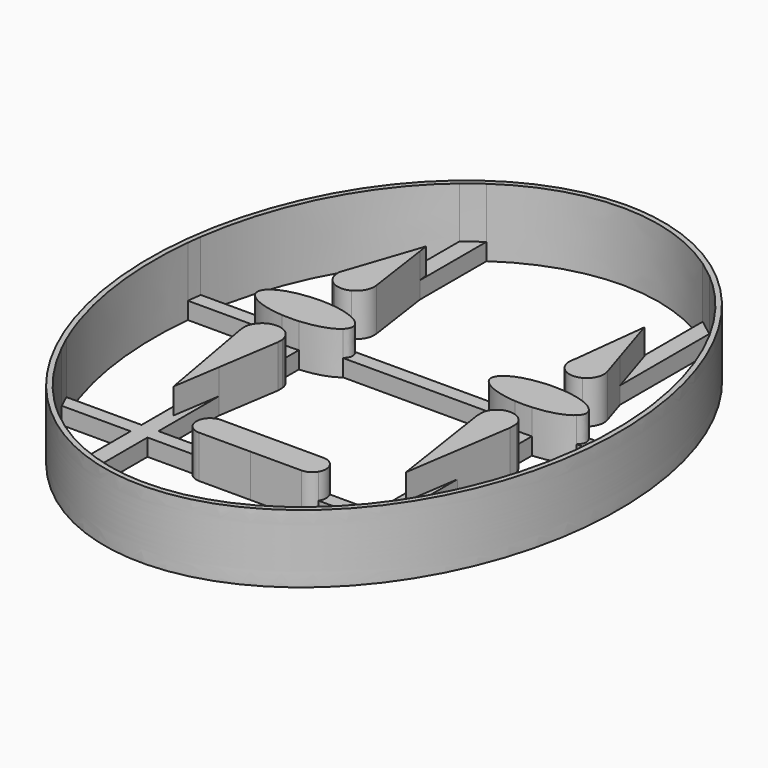
from build123d import *

# Parameters (mm, degrees)
F1_DEPTH = 10.16
F2_DEPTH = 6.35
F3_DEPTH = 2.54


# Not quite as in the source:
# - the dataset's text gives a spline's control points without its knots; the knots are read off the source's solid


with BuildPart() as f1:
    # F0 (on Top) → F1 (new body)
    with BuildSketch(Plane.XY):
        with BuildLine():
            add(Edge.make_bspline(
                [(0.8874152158, 46.7860518305), (0.3035465665, 46.7860518305), (-0.8641907321, 46.7484087934), (-3.1804804426, 46.524648738), (-6.0388714179, 45.9705936493), (-9.3828884747, 44.8801852683), (-12.6174065606, 43.3780630031), (-15.7189563215, 41.4780777699), (-18.6646785296, 39.1941395739), (-20.9712493188, 36.9817445808), (-22.7157476895, 35.0339858624), (-23.9729196354, 33.4833733883), (-25.1682601082, 31.8548035031), (-26.6676910685, 29.5980430053), (-28.3672543912, 26.6201447797), (-30.1171589074, 22.8270664956), (-31.5692954578, 18.84316303), (-32.7148026715, 14.6976460619), (-33.5447958259, 10.419700464), (-33.965961995, 6.767927242), (-34.135986765, 3.8102925283), (-34.1788837939, 1.5740518305), (-34.135986765, -0.6621888672), (-33.965961995, -3.619823581), (-33.5447958259, -7.271596803), (-32.7148026715, -11.5495424009), (-31.5692954578, -15.6950593689), (-30.1171589074, -19.6789628346), (-28.3672543912, -23.4720411187), (-26.6676910685, -26.4499393442), (-25.1682601082, -28.7066998421), (-23.9729196354, -30.3352697272), (-22.7157476895, -31.8858822014), (-20.9712493188, -33.8336409198), (-18.6646785296, -36.0460359129), (-15.7189563215, -38.3299741089), (-12.6174065606, -40.2299593421), (-9.3828884747, -41.7320816073), (-6.0388714179, -42.8224899883), (-3.1804804426, -43.376545077), (-0.8641907321, -43.6003051324), (0.8874152158, -43.656769688), (2.6390211637, -43.6003051324), (4.9553108741, -43.376545077), (7.8137018494, -42.8224899883), (11.1577189062, -41.7320816073), (14.3922369922, -40.2299593421), (17.493786753, -38.3299741089), (20.4395089612, -36.0460359129), (22.7460797504, -33.8336409198), (24.490578121, -31.8858822014), (25.7477500669, -30.3352697272), (26.9430905397, -28.7066998421), (28.4425215001, -26.4499393442), (30.1420848227, -23.4720411187), (31.8919893389, -19.6789628346), (33.3441258894, -15.6950593689), (34.489633103, -11.5495424009), (35.3196262574, -7.271596803), (35.7407924266, -3.619823581), (35.9108171965, -0.6621888672), (35.9537142254, 1.5740518305), (35.9108171965, 3.8102925283), (35.7407924266, 6.767927242), (35.3196262574, 10.419700464), (34.489633103, 14.6976460619), (33.3441258894, 18.84316303), (31.8919893389, 22.8270664956), (30.1420848227, 26.6201447797), (28.4425215001, 29.5980430053), (26.9430905397, 31.8548035031), (25.7477500669, 33.4833733883), (24.490578121, 35.0339858624), (22.7460797504, 36.9817445808), (20.4395089612, 39.1941395739), (17.493786753, 41.4780777699), (14.3922369922, 43.3780630031), (11.1577189062, 44.8801852683), (7.8137018494, 45.9705936493), (4.9553108741, 46.524648738), (2.6390211637, 46.7484087934), (1.4712838651, 46.7860518305), (0.8874152158, 46.7860518305)],
                knots=[0, 0, 0, 0, 0.0078125, 0.015625, 0.03125, 0.046875, 0.0625, 0.078125, 0.09375, 0.109375, 0.1171875, 0.125, 0.1328125, 0.140625, 0.15625, 0.171875, 0.1875, 0.203125, 0.21875, 0.234375, 0.2421875, 0.25, 0.2578125, 0.265625, 0.28125, 0.296875, 0.3125, 0.328125, 0.34375, 0.359375, 0.3671875, 0.375, 0.3828125, 0.390625, 0.40625, 0.421875, 0.4375, 0.453125, 0.46875, 0.484375, 0.4921875, 0.5, 0.5078125, 0.515625, 0.53125, 0.546875, 0.5625, 0.578125, 0.59375, 0.609375, 0.6171875, 0.625, 0.6328125, 0.640625, 0.65625, 0.671875, 0.6875, 0.703125, 0.71875, 0.734375, 0.7421875, 0.75, 0.7578125, 0.765625, 0.78125, 0.796875, 0.8125, 0.828125, 0.84375, 0.859375, 0.8671875, 0.875, 0.8828125, 0.890625, 0.90625, 0.921875, 0.9375, 0.953125, 0.96875, 0.984375, 0.9921875, 1, 1, 1, 1], degree=3))
        make_face()
        with BuildLine():
            add(Edge.make_bspline(
                [(0.8874152158, 46.0240518305), (-7.6730270574, 46.0240518305), (-15.2290235078, 40.8084782188)],
                knots=[0, 0, 0, 0.4892953614, 0.4892953614, 0.4892953614], degree=2, weights=[1, 0.970222722, 1]))
            add(Edge.make_bspline(
                [(17.0038539393, 40.8084782188), (9.447857489, 46.0240518305), (0.8874152158, 46.0240518305)],
                knots=[5.7938899458, 5.7938899458, 5.7938899458, 6.2831853072, 6.2831853072, 6.2831853072], degree=2, weights=[1, 0.970222722, 1]))
            add(Edge.make_bspline(
                [(19.5227909328, 38.8868294251), (18.2949402613, 39.9172978436), (17.0038539393, 40.8084782188)],
                knots=[5.7086272545, 5.7086272545, 5.7086272545, 5.7938899458, 5.7938899458, 5.7938899458], degree=2, weights=[1, 0.9990914218, 1]))
            add(Edge.make_bspline(
                [(34.6163309811, 9.5822196506), (31.9493168533, 28.457920756), (19.5227909328, 38.8868294251)],
                knots=[4.8935393675, 4.8935393675, 4.8935393675, 5.7086272545, 5.7086272545, 5.7086272545], degree=2, weights=[1, 0.9180970627, 1]))
            add(Edge.make_bspline(
                [(34.8708896875, 7.5041735472), (34.7625862899, 8.5471027136), (34.6163309811, 9.5822196506)],
                knots=[4.8461989994, 4.8461989994, 4.8461989994, 4.8935393675, 4.8935393675, 4.8935393675], degree=2, weights=[1, 0.9997198743, 1]))
            add(Edge.make_bspline(
                [(30.7375906283, -20.3011595258), (36.408100645, -7.2987059431), (34.8708896875, 7.5041735472)],
                knots=[4.1978532573, 4.1978532573, 4.1978532573, 4.8461989994, 4.8461989994, 4.8461989994], degree=2, weights=[1, 0.9479145118, 1]))
            add(Edge.make_bspline(
                [(29.7867641343, -22.3506663998), (30.2834517092, -21.3424979944), (30.7375906283, -20.3011595258)],
                knots=[4.1440428934, 4.1440428934, 4.1440428934, 4.1978532573, 4.1978532573, 4.1978532573], degree=2, weights=[1, 0.9996380774, 1]))
            add(Edge.make_bspline(
                [(19.5227909328, -35.7387257641), (25.7767590963, -30.490109762), (29.7867641343, -22.3506663998)],
                knots=[3.7161507062, 3.7161507062, 3.7161507062, 4.1440428934, 4.1440428934, 4.1440428934], degree=2, weights=[1, 0.9772006998, 1]))
            add(Edge.make_bspline(
                [(17.0038539393, -37.6603745577), (18.2949402613, -36.7691941826), (19.5227909328, -35.7387257641)],
                knots=[3.630888015, 3.630888015, 3.630888015, 3.7161507062, 3.7161507062, 3.7161507062], degree=2, weights=[1, 0.9990914218, 1]))
            add(Edge.make_bspline(
                [(-15.2290235078, -37.6603745577), (0.8874152158, -48.7848467666), (17.0038539393, -37.6603745577)],
                knots=[2.6522972922, 2.6522972922, 2.6522972922, 3.630888015, 3.630888015, 3.630888015], degree=2, weights=[1, 0.8826642607, 1]))
            add(Edge.make_bspline(
                [(-17.7479605013, -35.7387257641), (-16.5201098298, -36.7691941826), (-15.2290235078, -37.6603745577)],
                knots=[2.5670346009, 2.5670346009, 2.5670346009, 2.6522972922, 2.6522972922, 2.6522972922], degree=2, weights=[1, 0.9990914218, 1]))
            add(Edge.make_bspline(
                [(-28.0119337027, -22.3506663998), (-24.0019286648, -30.490109762), (-17.7479605013, -35.7387257641)],
                knots=[2.1391424138, 2.1391424138, 2.1391424138, 2.5670346009, 2.5670346009, 2.5670346009], degree=2, weights=[1, 0.9772006998, 1]))
            add(Edge.make_bspline(
                [(-28.9627601968, -20.3011595258), (-28.5086212776, -21.3424979944), (-28.0119337027, -22.3506663998)],
                knots=[2.0853320499, 2.0853320499, 2.0853320499, 2.1391424138, 2.1391424138, 2.1391424138], degree=2, weights=[1, 0.9996380774, 1]))
            add(Edge.make_bspline(
                [(-33.096059256, 7.5041735472), (-34.6332702135, -7.2987059431), (-28.9627601968, -20.3011595258)],
                knots=[1.4369863078, 1.4369863078, 1.4369863078, 2.0853320499, 2.0853320499, 2.0853320499], degree=2, weights=[1, 0.9479145118, 1]))
            add(Edge.make_bspline(
                [(-32.8415005495, 9.5822196506), (-32.9877558584, 8.5471027136), (-33.096059256, 7.5041735472)],
                knots=[1.3896459397, 1.3896459397, 1.3896459397, 1.4369863078, 1.4369863078, 1.4369863078], degree=2, weights=[1, 0.9997198743, 1]))
            add(Edge.make_bspline(
                [(-17.7479605013, 38.8868294251), (-30.1744864217, 28.457920756), (-32.8415005495, 9.5822196506)],
                knots=[0.5745580526, 0.5745580526, 0.5745580526, 1.3896459397, 1.3896459397, 1.3896459397], degree=2, weights=[1, 0.9180970627, 1]))
            add(Edge.make_bspline(
                [(-15.2290235078, 40.8084782188), (-16.5201098298, 39.9172978436), (-17.7479605013, 38.8868294251)],
                knots=[0.4892953614, 0.4892953614, 0.4892953614, 0.5745580526, 0.5745580526, 0.5745580526], degree=2, weights=[1, 0.9990914218, 1]))
        make_face(mode=Mode.SUBTRACT)
    extrude(amount=F1_DEPTH)



with BuildPart() as f2:
    # F0 (on Top) → F2 (new body)
    with BuildSketch(Plane.XY):
        with BuildLine():
            add(Edge.make_bspline(
                [(-17.7479605013, 11.44730103), (-21.8523231253, 11.159864588), (-23.2315880612, 9.5822196506)],
                knots=[4.88516773, 4.88516773, 4.88516773, 5.9457744715, 5.9457744715, 5.9457744715], degree=2, weights=[1, 0.8626536668, 1]))
            add(Edge.make_bspline(
                [(-23.2315880612, 9.5822196506), (-23.6322576844, 9.1239216208), (-23.6322576844, 8.6382383173)],
                knots=[5.9457744715, 5.9457744715, 5.9457744715, 6.2831853072, 6.2831853072, 6.2831853072], degree=2, weights=[1, 0.9858029614, 1]))
            add(Edge.make_bspline(
                [(-23.6322576844, 8.6382383173), (-23.6322576844, 8.0468135504), (-23.0461097972, 7.5041735472)],
                knots=[0, 0, 0, 0.4090146334, 0.4090146334, 0.4090146334], degree=2, weights=[1, 0.9791611598, 1]))
            add(Edge.make_bspline(
                [(-23.0461097972, 7.5041735472), (-21.522333432, 6.093502231), (-17.7479605013, 5.8291756045)],
                knots=[0.4090146334, 0.4090146334, 0.4090146334, 1.3980175772, 1.3980175772, 1.3980175772], degree=2, weights=[1, 0.8802054171, 1]))
            add(Edge.make_bspline(
                [(-17.7479605013, 5.8291756045), (-16.4872656687, 5.7408867104), (-15.2290235078, 5.8346406134)],
                knots=[1.3980175772, 1.3980175772, 1.3980175772, 1.7543880589, 1.7543880589, 1.7543880589], degree=2, weights=[1, 0.9841669681, 1]))
            add(Edge.make_bspline(
                [(-15.2290235078, 5.8346406134), (-11.5106062448, 6.1117066203), (-10.0064938636, 7.5041735472)],
                knots=[1.7543880589, 1.7543880589, 1.7543880589, 2.7325780202, 2.7325780202, 2.7325780202], degree=2, weights=[1, 0.8827584227, 1]))
            add(Edge.make_bspline(
                [(-10.0064938636, 7.5041735472), (-8.8999042079, 8.5286245899), (-9.8210155996, 9.5822196506)],
                knots=[2.7325780202, 2.7325780202, 2.7325780202, 3.4790034893, 3.4790034893, 3.4790034893], degree=2, weights=[1, 0.9311607616, 1]))
            add(Edge.make_bspline(
                [(-9.8210155996, 9.5822196506), (-11.1832439782, 11.1403776587), (-15.2290235078, 11.4418360212)],
                knots=[3.4790034893, 3.4790034893, 3.4790034893, 4.5287972483, 4.5287972483, 4.5287972483], degree=2, weights=[1, 0.8653756223, 1]))
            add(Edge.make_bspline(
                [(-15.2290235078, 11.4418360212), (-16.4872656687, 11.5355899242), (-17.7479605013, 11.44730103)],
                knots=[4.5287972483, 4.5287972483, 4.5287972483, 4.88516773, 4.88516773, 4.88516773], degree=2, weights=[1, 0.9841669681, 1]))
        make_face()
    extrude(amount=F2_DEPTH)


with BuildPart() as f2b:
    # F0 (on Top) → F2, piece 2 (new body)
    with BuildSketch(Plane.XY):
        with BuildLine():
            Line((-13.8026518037, 18.5152967152), (-15.2290235078, 28.4465199794))
            Line((-15.2290235078, 28.4465199794), (-15.4276108953, 29.8292000182))
            Line((-15.4276108953, 29.8292000182), (-17.7479605013, 22.9402716964))
            Line((-17.7479605013, 22.9402716964), (-19.2382517874, 18.5157186799))
            ThreePointArc((-19.2382517874, 18.5157186799), (-18.953046125, 16.8515255575), (-17.7479605013, 15.6688803622))
            ThreePointArc((-17.7479605013, 15.6688803622), (-16.4844803046, 15.3794653342), (-15.2290235078, 15.7019114496))
            ThreePointArc((-15.2290235078, 15.7019114496), (-14.0715265067, 16.8833406396), (-13.8026518037, 18.5152967152))
        make_face()
    extrude(amount=F2_DEPTH)


with BuildPart() as f2c:
    # F0 (on Top) → F2, piece 3 (new body)
    with BuildSketch(Plane.XY):
        with BuildLine():
            Line((17.1461113686, 29.7382220353), (17.0038539393, 28.497185345))
            Line((17.0038539393, 28.497185345), (15.8444382697, 18.382582593))
            ThreePointArc((15.8444382697, 18.382582593), (15.8857831263, 16.6578406118), (17.0038539393, 15.3439296727))
            ThreePointArc((17.0038539393, 15.3439296727), (18.2581575627, 14.9961423132), (19.5227909328, 15.3042592817))
            ThreePointArc((19.5227909328, 15.3042592817), (20.6927393028, 16.6091812711), (20.7603491707, 18.3604749337))
            Line((20.7603491707, 18.3604749337), (19.5227909328, 22.2563515817))
            Line((19.5227909328, 22.2563515817), (17.1461113686, 29.7382220353))
        make_face()
    extrude(amount=F2_DEPTH)


with BuildPart() as f2d:
    # F0 (on Top) → F2, piece 4 (new body)
    with BuildSketch(Plane.XY):
        with BuildLine():
            add(Edge.make_bspline(
                [(25.4135646224, 8.6382383173), (25.4135646224, 9.1239216208), (25.0128949991, 9.5822196506)],
                knots=[0, 0, 0, 0.3374108357, 0.3374108357, 0.3374108357], degree=2, weights=[1, 0.9858029614, 1]))
            add(Edge.make_bspline(
                [(25.0128949991, 9.5822196506), (23.632167473, 11.1615375429), (19.5227909328, 11.4477533536)],
                knots=[0.3374108357, 0.3374108357, 0.3374108357, 1.3989426975, 1.3989426975, 1.3989426975], degree=2, weights=[1, 0.8624196139, 1]))
            add(Edge.make_bspline(
                [(19.5227909328, 11.4477533536), (18.2618860231, 11.5355746855), (17.0038539393, 11.4413521986)],
                knots=[1.3989426975, 1.3989426975, 1.3989426975, 1.7553151371, 1.7553151371, 1.7553151371], degree=2, weights=[1, 0.9841667946, 1]))
            add(Edge.make_bspline(
                [(17.0038539393, 11.4413521986), (12.9630952221, 11.1387125918), (11.6023225375, 9.5822196506)],
                knots=[1.7553151371, 1.7553151371, 1.7553151371, 2.8041818179, 2.8041818179, 2.8041818179], degree=2, weights=[1, 0.8656078198, 1]))
            add(Edge.make_bspline(
                [(11.6023225375, 9.5822196506), (10.6812111458, 8.5286245899), (11.7878008015, 7.5041735472)],
                knots=[2.8041818179, 2.8041818179, 2.8041818179, 3.5506072869, 3.5506072869, 3.5506072869], degree=2, weights=[1, 0.9311607616, 1]))
            add(Edge.make_bspline(
                [(11.7878008015, 7.5041735472), (13.2902325239, 6.1132625292), (17.0038539393, 5.8351244359)],
                knots=[3.5506072869, 3.5506072869, 3.5506072869, 4.5278701701, 4.5278701701, 4.5278701701], degree=2, weights=[1, 0.8829761111, 1]))
            add(Edge.make_bspline(
                [(17.0038539393, 5.8351244359), (18.2618860231, 5.7409019491), (19.5227909328, 5.828723281)],
                knots=[4.5278701701, 4.5278701701, 4.5278701701, 4.8842426097, 4.8842426097, 4.8842426097], degree=2, weights=[1, 0.9841667946, 1]))
            add(Edge.make_bspline(
                [(19.5227909328, 5.828723281), (23.3019526806, 6.0919398134), (24.8274167351, 7.5041735472)],
                knots=[4.8842426097, 4.8842426097, 4.8842426097, 5.8741706738, 5.8741706738, 5.8741706738], degree=2, weights=[1, 0.8799857952, 1]))
            add(Edge.make_bspline(
                [(24.8274167351, 7.5041735472), (25.4135646224, 8.0468135504), (25.4135646224, 8.6382383173)],
                knots=[5.8741706738, 5.8741706738, 5.8741706738, 6.2831853072, 6.2831853072, 6.2831853072], degree=2, weights=[1, 0.9791611598, 1]))
        make_face()
    extrude(amount=F2_DEPTH)


with BuildPart() as f2e:
    # F0 (on Top) → F2, piece 5 (new body)
    with BuildSketch(Plane.XY):
        with BuildLine():
            Line((18.3088215866, -16.1279799693), (19.5227909328, -8.0577728991))
            Line((19.5227909328, -8.0577728991), (20.7629566947, 0.1865823074))
            Line((20.7629566947, 0.1865823074), (20.7627794612, 1.4218628216))
            ThreePointArc((20.7627794612, 1.4218628216), (20.3102626812, 2.3535523253), (19.5227909328, 3.0263858953))
            ThreePointArc((19.5227909328, 3.0263858953), (18.9347962572, 3.2586504045), (18.3076087683, 3.3381513144))
            Line((18.3076087683, 3.3381513144), (18.3023937202, 3.3381513144))
            ThreePointArc((18.3023937202, 3.3381513144), (17.6287933652, 3.2462728126), (17.0038539393, 2.9786353503))
            ThreePointArc((17.0038539393, 2.9786353503), (16.2672974346, 2.3106387051), (15.8444382697, 1.4106803009))
            Line((15.8444382697, 1.4106803009), (15.8444382697, 0.1970595365))
            Line((15.8444382697, 0.1970595365), (17.0038539393, -7.4833635861))
            Line((17.0038539393, -7.4833635861), (18.3088215866, -16.1279799693))
        make_face()
    extrude(amount=F2_DEPTH)


with BuildPart() as f2f:
    # F0 (on Top) → F2, piece 6 (new body)
    with BuildSketch(Plane.XY):
        with BuildLine():
            Line((-19.2441018304, 0.1865863317), (-17.7479605013, -8.1779694256))
            Line((-17.7479605013, -8.1779694256), (-16.3255312883, -16.1304189912))
            Line((-16.3255312883, -16.1304189912), (-15.2290235078, -9.0221496637))
            Line((-15.2290235078, -9.0221496637), (-13.8085018304, 0.1865863317))
            Line((-13.8085018304, 0.1865863317), (-13.8085018304, 1.0250714))
            ThreePointArc((-13.8085018304, 1.0250714), (-14.2822654949, 2.195326292), (-15.2290235078, 3.0305494881))
            ThreePointArc((-15.2290235078, 3.0305494881), (-15.7076702442, 3.2310990364), (-16.2154720062, 3.3381513144))
            Line((-16.2154720062, 3.3381513144), (-16.5263018304, 3.3381513144))
            Line((-16.5263018304, 3.3381513144), (-16.8371316545, 3.3381513144))
            ThreePointArc((-16.8371316545, 3.3381513144), (-17.304229567, 3.2434470298), (-17.7479605013, 3.0695153788))
            ThreePointArc((-17.7479605013, 3.0695153788), (-18.745484439, 2.2298453965), (-19.2441018304, 1.0250714))
            Line((-19.2441018304, 1.0250714), (-19.2441018304, 0.1865863317))
        make_face()
    extrude(amount=F2_DEPTH)


with BuildPart() as f2g:
    # F0 (on Top) → F2, piece 7 (new body)
    with BuildSketch(Plane.XY):
        with BuildLine():
            ThreePointArc((-8.5105954788, -20.3011595258), (-8.7762969648, -21.3283492866), (-8.4924240981, -22.3506663998))
            ThreePointArc((-8.4924240981, -22.3506663998), (-7.7440409154, -23.088748383), (-6.7281162348, -23.3584508958))
            Line((-6.7281162348, -23.3584508958), (0.8933992052, -23.3584508958))
            Line((0.8933992052, -23.3584508958), (8.5133986834, -23.355631034))
            ThreePointArc((8.5133986834, -23.355631034), (9.527123423, -23.0865386285), (10.2744791839, -22.3506663998))
            ThreePointArc((10.2744791839, -22.3506663998), (10.5593969681, -21.3285723586), (10.2942984138, -20.3011595258))
            ThreePointArc((10.2942984138, -20.3011595258), (9.5436122613, -19.5405321417), (8.5118837652, -19.2619284317))
            Line((8.5118837652, -19.2619284317), (0.8918837652, -19.2619284317))
            Line((0.8918837652, -19.2619284317), (-6.7281162348, -19.2619284317))
            ThreePointArc((-6.7281162348, -19.2619284317), (-7.7597694616, -19.5407079051), (-8.5105954788, -20.3011595258))
        make_face()
    extrude(amount=F2_DEPTH)


with BuildPart() as f1_1:
    add(f1.part)

    add(f2.part)  # F3 merges F2

    add(f2b.part)  # F3 merges F2b

    add(f2c.part)  # F3 merges F2c

    add(f2d.part)  # F3 merges F2d

    add(f2e.part)  # F3 merges F2e

    add(f2f.part)  # F3 merges F2f

    add(f2g.part)  # F3 merges F2g
    # F0 (on Top) → F3 (join)
    with BuildSketch(Plane.XY):
        with BuildLine():
            ThreePointArc((19.5227909328, 15.3042592817), (18.2581575627, 14.9961423132), (17.0038539393, 15.3439296727))
            Line((17.0038539393, 15.3439296727), (17.0038539393, 11.4413521986))
            add(Edge.make_bspline(
                [(19.5227909328, 11.4477533536), (18.2618860231, 11.5355746855), (17.0038539393, 11.4413521986)],
                knots=[1.3989426975, 1.3989426975, 1.3989426975, 1.7553151371, 1.7553151371, 1.7553151371], degree=2, weights=[1, 0.9841667946, 1]))
            Line((19.5227909328, 11.4477533536), (19.5227909328, 15.3042592817))
        make_face()
        with BuildLine():
            add(Edge.make_bspline(
                [(34.8708896875, 7.5041735472), (34.7625862899, 8.5471027136), (34.6163309811, 9.5822196506)],
                knots=[4.8461989994, 4.8461989994, 4.8461989994, 4.8935393675, 4.8935393675, 4.8935393675], degree=2, weights=[1, 0.9997198743, 1]))
            Line((34.6163309811, 9.5822196506), (25.0128949991, 9.5822196506))
            add(Edge.make_bspline(
                [(25.4135646224, 8.6382383173), (25.4135646224, 9.1239216208), (25.0128949991, 9.5822196506)],
                knots=[0, 0, 0, 0.3374108357, 0.3374108357, 0.3374108357], degree=2, weights=[1, 0.9858029614, 1]))
            add(Edge.make_bspline(
                [(24.8274167351, 7.5041735472), (25.4135646224, 8.0468135504), (25.4135646224, 8.6382383173)],
                knots=[5.8741706738, 5.8741706738, 5.8741706738, 6.2831853072, 6.2831853072, 6.2831853072], degree=2, weights=[1, 0.9791611598, 1]))
            Line((24.8274167351, 7.5041735472), (34.8708896875, 7.5041735472))
        make_face()
        with BuildLine():
            Line((11.6023225375, 9.5822196506), (-9.8210155996, 9.5822196506))
            add(Edge.make_bspline(
                [(-10.0064938636, 7.5041735472), (-8.8999042079, 8.5286245899), (-9.8210155996, 9.5822196506)],
                knots=[2.7325780202, 2.7325780202, 2.7325780202, 3.4790034893, 3.4790034893, 3.4790034893], degree=2, weights=[1, 0.9311607616, 1]))
            Line((-10.0064938636, 7.5041735472), (11.7878008015, 7.5041735472))
            add(Edge.make_bspline(
                [(11.6023225375, 9.5822196506), (10.6812111458, 8.5286245899), (11.7878008015, 7.5041735472)],
                knots=[2.8041818179, 2.8041818179, 2.8041818179, 3.5506072869, 3.5506072869, 3.5506072869], degree=2, weights=[1, 0.9311607616, 1]))
        make_face()
        with BuildLine():
            Line((19.5227909328, 3.0263858953), (19.5227909328, 5.828723281))
            add(Edge.make_bspline(
                [(17.0038539393, 5.8351244359), (18.2618860231, 5.7409019491), (19.5227909328, 5.828723281)],
                knots=[4.5278701701, 4.5278701701, 4.5278701701, 4.8842426097, 4.8842426097, 4.8842426097], degree=2, weights=[1, 0.9841667946, 1]))
            Line((17.0038539393, 5.8351244359), (17.0038539393, 2.9786353503))
            ThreePointArc((17.0038539393, 2.9786353503), (17.6287933652, 3.2462728126), (18.3023937202, 3.3381513144))
            Line((18.3023937202, 3.3381513144), (18.3076087683, 3.3381513144))
            ThreePointArc((18.3076087683, 3.3381513144), (18.9347962572, 3.2586504045), (19.5227909328, 3.0263858953))
        make_face()
        with BuildLine():
            add(Edge.make_bspline(
                [(29.7867641343, -22.3506663998), (30.2834517092, -21.3424979944), (30.7375906283, -20.3011595258)],
                knots=[4.1440428934, 4.1440428934, 4.1440428934, 4.1978532573, 4.1978532573, 4.1978532573], degree=2, weights=[1, 0.9996380774, 1]))
            Line((30.7375906283, -20.3011595258), (19.5227909328, -20.3011595258))
            Line((19.5227909328, -20.3011595258), (19.5227909328, -8.0577728991))
            Line((19.5227909328, -8.0577728991), (18.3088215866, -16.1279799693))
            Line((18.3088215866, -16.1279799693), (17.0038539393, -7.4833635861))
            Line((17.0038539393, -7.4833635861), (17.0038539393, -20.3011595258))
            Line((17.0038539393, -20.3011595258), (10.2942984138, -20.3011595258))
            ThreePointArc((10.2942984138, -20.3011595258), (10.5593969681, -21.3285723586), (10.2744791839, -22.3506663998))
            Line((10.2744791839, -22.3506663998), (17.0038539393, -22.3506663998))
            Line((17.0038539393, -22.3506663998), (17.0038539393, -37.6603745577))
            add(Edge.make_bspline(
                [(17.0038539393, -37.6603745577), (18.2949402613, -36.7691941826), (19.5227909328, -35.7387257641)],
                knots=[3.630888015, 3.630888015, 3.630888015, 3.7161507062, 3.7161507062, 3.7161507062], degree=2, weights=[1, 0.9990914218, 1]))
            Line((19.5227909328, -35.7387257641), (19.5227909328, -22.3506663998))
            Line((19.5227909328, -22.3506663998), (29.7867641343, -22.3506663998))
        make_face()
        with BuildLine():
            Line((-17.7479605013, -20.3011595258), (-28.9627601968, -20.3011595258))
            add(Edge.make_bspline(
                [(-28.9627601968, -20.3011595258), (-28.5086212776, -21.3424979944), (-28.0119337027, -22.3506663998)],
                knots=[2.0853320499, 2.0853320499, 2.0853320499, 2.1391424138, 2.1391424138, 2.1391424138], degree=2, weights=[1, 0.9996380774, 1]))
            Line((-28.0119337027, -22.3506663998), (-17.7479605013, -22.3506663998))
            Line((-17.7479605013, -22.3506663998), (-17.7479605013, -35.7387257641))
            add(Edge.make_bspline(
                [(-17.7479605013, -35.7387257641), (-16.5201098298, -36.7691941826), (-15.2290235078, -37.6603745577)],
                knots=[2.5670346009, 2.5670346009, 2.5670346009, 2.6522972922, 2.6522972922, 2.6522972922], degree=2, weights=[1, 0.9990914218, 1]))
            Line((-15.2290235078, -37.6603745577), (-15.2290235078, -22.3506663998))
            Line((-15.2290235078, -22.3506663998), (-8.4924240981, -22.3506663998))
            ThreePointArc((-8.4924240981, -22.3506663998), (-8.7762969648, -21.3283492866), (-8.5105954788, -20.3011595258))
            Line((-8.5105954788, -20.3011595258), (-15.2290235078, -20.3011595258))
            Line((-15.2290235078, -20.3011595258), (-15.2290235078, -9.0221496637))
            Line((-15.2290235078, -9.0221496637), (-16.3255312883, -16.1304189912))
            Line((-16.3255312883, -16.1304189912), (-17.7479605013, -8.1779694256))
            Line((-17.7479605013, -8.1779694256), (-17.7479605013, -20.3011595258))
        make_face()
        with BuildLine():
            Line((-23.2315880612, 9.5822196506), (-32.8415005495, 9.5822196506))
            add(Edge.make_bspline(
                [(-32.8415005495, 9.5822196506), (-32.9877558584, 8.5471027136), (-33.096059256, 7.5041735472)],
                knots=[1.3896459397, 1.3896459397, 1.3896459397, 1.4369863078, 1.4369863078, 1.4369863078], degree=2, weights=[1, 0.9997198743, 1]))
            Line((-33.096059256, 7.5041735472), (-23.0461097972, 7.5041735472))
            add(Edge.make_bspline(
                [(-23.6322576844, 8.6382383173), (-23.6322576844, 8.0468135504), (-23.0461097972, 7.5041735472)],
                knots=[0, 0, 0, 0.4090146334, 0.4090146334, 0.4090146334], degree=2, weights=[1, 0.9791611598, 1]))
            add(Edge.make_bspline(
                [(-23.2315880612, 9.5822196506), (-23.6322576844, 9.1239216208), (-23.6322576844, 8.6382383173)],
                knots=[5.9457744715, 5.9457744715, 5.9457744715, 6.2831853072, 6.2831853072, 6.2831853072], degree=2, weights=[1, 0.9858029614, 1]))
        make_face()
        with BuildLine():
            add(Edge.make_bspline(
                [(-17.7479605013, 5.8291756045), (-16.4872656687, 5.7408867104), (-15.2290235078, 5.8346406134)],
                knots=[1.3980175772, 1.3980175772, 1.3980175772, 1.7543880589, 1.7543880589, 1.7543880589], degree=2, weights=[1, 0.9841669681, 1]))
            Line((-17.7479605013, 5.8291756045), (-17.7479605013, 3.0695153788))
            ThreePointArc((-17.7479605013, 3.0695153788), (-17.304229567, 3.2434470298), (-16.8371316545, 3.3381513144))
            ThreePointArc((-16.8371316545, 3.3381513144), (-16.6819663392, 3.3513651892), (-16.5263018304, 3.3557745276))
            ThreePointArc((-16.5263018304, 3.3557745276), (-16.3706373216, 3.3513651892), (-16.2154720062, 3.3381513144))
            ThreePointArc((-16.2154720062, 3.3381513144), (-15.7076702442, 3.2310990364), (-15.2290235078, 3.0305494881))
            Line((-15.2290235078, 3.0305494881), (-15.2290235078, 5.8346406134))
        make_face()
        with BuildLine():
            Line((-15.2290235078, 11.4418360212), (-15.2290235078, 15.7019114496))
            ThreePointArc((-15.2290235078, 15.7019114496), (-16.4844803046, 15.3794653342), (-17.7479605013, 15.6688803622))
            Line((-17.7479605013, 15.6688803622), (-17.7479605013, 11.44730103))
            add(Edge.make_bspline(
                [(-15.2290235078, 11.4418360212), (-16.4872656687, 11.5355899242), (-17.7479605013, 11.44730103)],
                knots=[4.5287972483, 4.5287972483, 4.5287972483, 4.88516773, 4.88516773, 4.88516773], degree=2, weights=[1, 0.9841669681, 1]))
        make_face()
        with BuildLine():
            add(Edge.make_bspline(
                [(19.5227909328, 38.8868294251), (18.2949402613, 39.9172978436), (17.0038539393, 40.8084782188)],
                knots=[5.7086272545, 5.7086272545, 5.7086272545, 5.7938899458, 5.7938899458, 5.7938899458], degree=2, weights=[1, 0.9990914218, 1]))
            Line((17.0038539393, 40.8084782188), (17.0038539393, 28.497185345))
            Line((17.0038539393, 28.497185345), (17.1461113686, 29.7382220353))
            Line((17.1461113686, 29.7382220353), (19.5227909328, 22.2563515817))
            Line((19.5227909328, 22.2563515817), (19.5227909328, 38.8868294251))
        make_face()
        with BuildLine():
            Line((-15.2290235078, 28.4465199794), (-15.2290235078, 40.8084782188))
            add(Edge.make_bspline(
                [(-15.2290235078, 40.8084782188), (-16.5201098298, 39.9172978436), (-17.7479605013, 38.8868294251)],
                knots=[0.4892953614, 0.4892953614, 0.4892953614, 0.5745580526, 0.5745580526, 0.5745580526], degree=2, weights=[1, 0.9990914218, 1]))
            Line((-17.7479605013, 38.8868294251), (-17.7479605013, 22.9402716964))
            Line((-17.7479605013, 22.9402716964), (-15.4276108953, 29.8292000182))
            Line((-15.4276108953, 29.8292000182), (-15.2290235078, 28.4465199794))
        make_face()
    extrude(amount=F3_DEPTH)


solid = f1_1.part
